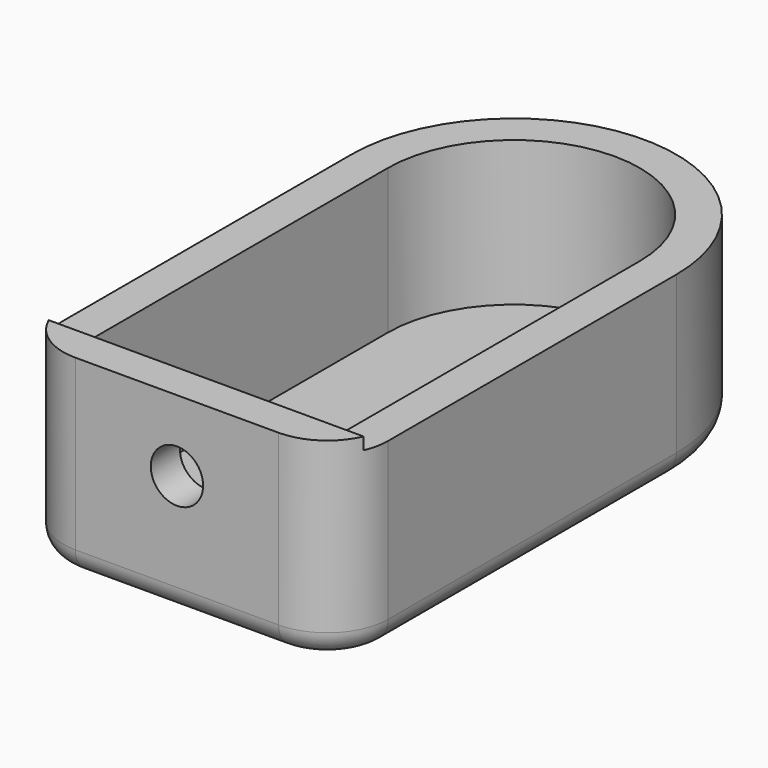
from build123d import *

# Parameters (mm, degrees)
F1_DEPTH    = 3
F2_DEPTH    = 11.9
F4_DEPTH    = 1
F6_DEPTH    = 6
F7_T1_DEPTH = 40.9
F8_R        = 2
F9_R        = 3.5272638361
F10_DEPTH   = 1
F11_DEPTH   = 25


# Not quite as in the source:
# - a fillet or chamfer that OpenCascade refuses, or shapes differently, is made with other operations: its cross-section is extruded or revolved along the edge and cut away or added


with BuildPart() as f1:
    # F0 (on Top) → F1 (new body)
    with BuildSketch(Plane.XY):
        with BuildLine():
            Line((13.35, -34.6), (13.35, 0))
            ThreePointArc((13.35, 0), (0, 13.35), (-13.35, 0))
            Line((-13.35, 0), (-13.35, -34.6))
            Line((-13.35, -34.6), (13.35, -34.6))
        make_face()
        with BuildLine():
            Line((-10.35, -31.6), (-10.35, 0))
            ThreePointArc((-10.35, 0), (0, 10.35), (10.35, 0))
            Line((10.35, 0), (10.35, -31.6))
            Line((10.35, -31.6), (-10.35, -31.6))
        make_face(mode=Mode.SUBTRACT)
        with BuildLine():
            ThreePointArc((10.35, 0), (0, 10.35), (-10.35, 0))
            Line((-10.35, 0), (-10.35, -31.6))
            Line((-10.35, -31.6), (10.35, -31.6))
            Line((10.35, -31.6), (10.35, 0))
        make_face()
    extrude(amount=-F1_DEPTH)

    # F0 (on Top) → F2 (join)
    with BuildSketch(Plane.XY):
        with BuildLine():
            Line((13.35, -34.6), (13.35, 0))
            ThreePointArc((13.35, 0), (0, 13.35), (-13.35, 0))
            Line((-13.35, 0), (-13.35, -34.6))
            Line((-13.35, -34.6), (13.35, -34.6))
        make_face()
        with BuildLine():
            Line((-10.35, -31.6), (-10.35, 0))
            ThreePointArc((-10.35, 0), (0, 10.35), (10.35, 0))
            Line((10.35, 0), (10.35, -31.6))
            Line((10.35, -31.6), (-10.35, -31.6))
        make_face(mode=Mode.SUBTRACT)
    extrude(amount=F2_DEPTH)

    # F3 (on face) → F4 (join)
    with BuildSketch(Plane.XY.offset(11.9)):
        Polygon((-13.35, -34.6), (13.35, -34.6), (13.35, -31.6), (10.35, -31.6), (-10.35, -31.6), (-13.35, -31.6), align=None)
    extrude(amount=F4_DEPTH)

    # F5 (on face) → F6 (cut)
    with BuildSketch(Plane.XZ.offset(34.6)):
        with BuildLine():
            ThreePointArc((0, 9.2), (-2.15, 7.05), (0, 4.9))
            Line((0, 4.9), (0, 9.2))
        make_face()
        with BuildLine():
            Line((0, 9.2), (0, 4.9))
            ThreePointArc((0, 4.9), (1.5202795796, 5.5297204204), (2.15, 7.05))
            ThreePointArc((2.15, 7.05), (1.5202795796, 8.5702795796), (0, 9.2))
        make_face()
    extrude(amount=-F6_DEPTH, mode=Mode.SUBTRACT)

    # F7: fillet of radius 5 on 2 edges, made by hand

    # F7_s2 → F7_t1 (cut)
    with BuildSketch(Plane.XY.offset(-15.5)):
        with BuildLine():
            ThreePointArc((-13.35, -29.6), (-11.8855339059, -33.1355339059), (-8.35, -34.6))
            Line((-8.35, -34.6), (-13.35, -34.6))
            Line((-13.35, -34.6), (-13.35, -29.6))
        make_face()
        with BuildLine():
            ThreePointArc((8.35, -34.6), (11.8855339059, -33.1355339059), (13.35, -29.6))
            Line((13.35, -29.6), (13.35, -34.6))
            Line((13.35, -34.6), (8.35, -34.6))
        make_face()
    extrude(amount=F7_T1_DEPTH, mode=Mode.SUBTRACT)

    # F8
    f8_edges = [f1.edges().sort_by_distance(p)[0] for p in [
        (13.35, -14.8, -3),
    ]]
    fillet(f8_edges, radius=F8_R)

    # F9 (on face) → F10 (join)
    with BuildSketch(Plane(origin=(0, -31.6, 0), x_dir=(-1, 0, 0), z_dir=(0, 1, 0))):
        with Locations((0, 7.05)):
            Circle(F9_R)
    extrude(amount=-F10_DEPTH)

    # F11 (cut): a face of the model
    f11_faces = [f1.faces().sort_by_distance(p)[0] for p in [
        (0, -32.6, 7.05),
    ]]
    extrude(f11_faces, amount=-F11_DEPTH, mode=Mode.SUBTRACT)


solid = f1.part
